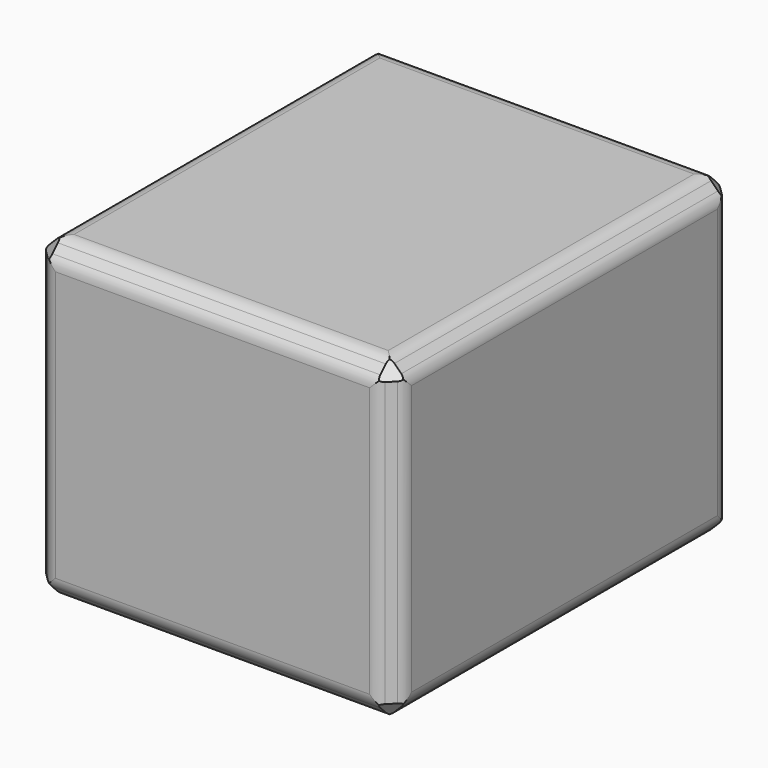
from build123d import *

# Parameters (mm, degrees)
F0_W        = 111.1548654735
F0_H        = 97.4772460759
F1_DEPTH    = 132.08
F2_SIZE     = 5.08
F3_T1_DEPTH = 132.4410244843
F3_T3_DEPTH = 111.5158899578
F3_T5_DEPTH = 97.8382705601


# Not quite as in the source:
# - a fillet or chamfer that OpenCascade refuses, or shapes differently, is made with other operations: its cross-section is extruded or revolved along the edge and cut away or added


with BuildPart() as f1:
    # F0 (on Front) → F1 (new body)
    with BuildSketch(Plane.XZ):
        with Locations((-0.1736786216, 1.3392996043)):
            Rectangle(F0_W, F0_H)
    extrude(amount=F1_DEPTH)

    # F2
    f2_edges = [f1.edges().sort_by_distance(p)[0] for p in [
        (55.403754, -66.04, 50.077923),
        (-55.751111, -66.04, 50.077923),
        (-0.173679, 0, 50.077923),
        (-0.173679, -132.08, 50.077923),
        (55.403754, -66.04, -47.399323),
        (55.403754, 0, 1.3393),
        (55.403754, -132.08, 1.3393),
        (-55.751111, -132.08, 1.3393),
        (-0.173679, -132.08, -47.399323),
        (-55.751111, -66.04, -47.399323),
        (-0.173679, 0, -47.399323),
        (-55.751111, 0, 1.3393),
    ]]
    chamfer(f2_edges, length=F2_SIZE)

    # F3: fillet of radius 5.08 on 24 edges, made by hand

    # F3_s2 → F3_t1 (cut)
    with BuildSketch(Plane.XZ.offset(-0.1805122421)):
        with BuildLine():
            ThreePointArc((48.2195492182, 50.0779226422), (50.1635810547, 49.6912306674), (51.8116516667, 48.5900250907))
            Line((51.8116516667, 48.5900250907), (50.3237541151, 50.0779226422))
            Line((50.3237541151, 50.0779226422), (48.2195492182, 50.0779226422))
        make_face()
        with BuildLine():
            ThreePointArc((-48.5669064615, 50.0779226422), (-50.510938298, 49.6912306674), (-52.15900891, 48.5900250907))
            Line((-52.15900891, 48.5900250907), (-50.6711113584, 50.0779226422))
            Line((-50.6711113584, 50.0779226422), (-48.5669064615, 50.0779226422))
        make_face()
        with BuildLine():
            ThreePointArc((53.9158565635, 46.4858201938), (55.0170621403, 44.8377495818), (55.4037541151, 42.8937177454))
            Line((55.4037541151, 42.8937177454), (55.4037541151, 44.9979226422))
            Line((55.4037541151, 44.9979226422), (53.9158565635, 46.4858201938))
        make_face()
        with BuildLine():
            ThreePointArc((55.4037541151, -40.2151185368), (55.0170621403, -42.1591503732), (53.9158565635, -43.8072209852))
            Line((53.9158565635, -43.8072209852), (55.4037541151, -42.3193234336))
            Line((55.4037541151, -42.3193234336), (55.4037541151, -40.2151185368))
        make_face()
        with BuildLine():
            ThreePointArc((51.8116516667, -45.9114258821), (50.1635810547, -47.0126314588), (48.2195492182, -47.3993234336))
            Line((48.2195492182, -47.3993234336), (50.3237541151, -47.3993234336))
            Line((50.3237541151, -47.3993234336), (51.8116516667, -45.9114258821))
        make_face()
        with BuildLine():
            ThreePointArc((-52.15900891, -45.9114258821), (-50.510938298, -47.0126314588), (-48.5669064615, -47.3993234336))
            Line((-48.5669064615, -47.3993234336), (-50.6711113584, -47.3993234336))
            Line((-50.6711113584, -47.3993234336), (-52.15900891, -45.9114258821))
        make_face()
        with BuildLine():
            ThreePointArc((-54.2632138068, 46.4858201938), (-55.3644193836, 44.8377495818), (-55.7511113584, 42.8937177454))
            Line((-55.7511113584, 42.8937177454), (-55.7511113584, 44.9979226422))
            Line((-55.7511113584, 44.9979226422), (-54.2632138068, 46.4858201938))
        make_face()
        with BuildLine():
            ThreePointArc((-55.7511113584, -40.2151185368), (-55.3644193836, -42.1591503732), (-54.2632138068, -43.8072209852))
            Line((-54.2632138068, -43.8072209852), (-55.7511113584, -42.3193234336))
            Line((-55.7511113584, -42.3193234336), (-55.7511113584, -40.2151185368))
        make_face()
    extrude(amount=F3_T1_DEPTH, mode=Mode.SUBTRACT)

    # F3_s4 → F3_t3 (cut)
    with BuildSketch(Plane.YZ.offset(-55.9316236005)):
        with BuildLine():
            ThreePointArc((-7.1842048969, 50.0779226422), (-5.2401730604, 49.6912306674), (-3.5921024484, 48.5900250907))
            Line((-3.5921024484, 48.5900250907), (-5.08, 50.0779226422))
            Line((-5.08, 50.0779226422), (-7.1842048969, 50.0779226422))
        make_face()
        with BuildLine():
            ThreePointArc((-124.8957951031, 50.0779226422), (-126.8398269396, 49.6912306674), (-128.4878975516, 48.5900250907))
            Line((-128.4878975516, 48.5900250907), (-127, 50.0779226422))
            Line((-127, 50.0779226422), (-124.8957951031, 50.0779226422))
        make_face()
        with BuildLine():
            ThreePointArc((-1.4878975516, 46.4858201938), (-0.3866919748, 44.8377495818), (0, 42.8937177454))
            Line((0, 42.8937177454), (0, 44.9979226422))
            Line((0, 44.9979226422), (-1.4878975516, 46.4858201938))
        make_face()
        with BuildLine():
            ThreePointArc((0, -40.2151185368), (-0.3866919748, -42.1591503732), (-1.4878975516, -43.8072209852))
            Line((-1.4878975516, -43.8072209852), (0, -42.3193234336))
            Line((0, -42.3193234336), (0, -40.2151185368))
        make_face()
        with BuildLine():
            ThreePointArc((-3.5921024484, -45.9114258821), (-5.2401730604, -47.0126314588), (-7.1842048969, -47.3993234336))
            Line((-7.1842048969, -47.3993234336), (-5.08, -47.3993234336))
            Line((-5.08, -47.3993234336), (-3.5921024484, -45.9114258821))
        make_face()
        with BuildLine():
            ThreePointArc((-128.4878975516, -45.9114258821), (-126.8398269396, -47.0126314588), (-124.8957951031, -47.3993234336))
            Line((-124.8957951031, -47.3993234336), (-127, -47.3993234336))
            Line((-127, -47.3993234336), (-128.4878975516, -45.9114258821))
        make_face()
        with BuildLine():
            ThreePointArc((-130.5921024484, 46.4858201938), (-131.6933080252, 44.8377495818), (-132.08, 42.8937177454))
            Line((-132.08, 42.8937177454), (-132.08, 44.9979226422))
            Line((-132.08, 44.9979226422), (-130.5921024484, 46.4858201938))
        make_face()
        with BuildLine():
            ThreePointArc((-132.08, -40.2151185368), (-131.6933080252, -42.1591503732), (-130.5921024484, -43.8072209852))
            Line((-130.5921024484, -43.8072209852), (-132.08, -42.3193234336))
            Line((-132.08, -42.3193234336), (-132.08, -40.2151185368))
        make_face()
    extrude(amount=F3_T3_DEPTH, mode=Mode.SUBTRACT)

    # F3_s6 → F3_t5 (cut)
    with BuildSketch(Plane.XY.offset(-47.5798356758)):
        with BuildLine():
            ThreePointArc((48.2195492182, 0), (50.1635810547, -0.3866919748), (51.8116516667, -1.4878975516))
            Line((51.8116516667, -1.4878975516), (50.3237541151, 0))
            Line((50.3237541151, 0), (48.2195492182, 0))
        make_face()
        with BuildLine():
            ThreePointArc((-48.5669064615, 0), (-50.510938298, -0.3866919748), (-52.15900891, -1.4878975516))
            Line((-52.15900891, -1.4878975516), (-50.6711113584, 0))
            Line((-50.6711113584, 0), (-48.5669064615, 0))
        make_face()
        with BuildLine():
            ThreePointArc((55.4037541151, -7.1842048969), (55.0170621403, -5.2401730604), (53.9158565635, -3.5921024484))
            Line((53.9158565635, -3.5921024484), (55.4037541151, -5.08))
            Line((55.4037541151, -5.08), (55.4037541151, -7.1842048969))
        make_face()
        with BuildLine():
            ThreePointArc((55.4037541151, -124.8957951031), (55.0170621403, -126.8398269396), (53.9158565635, -128.4878975516))
            Line((53.9158565635, -128.4878975516), (55.4037541151, -127))
            Line((55.4037541151, -127), (55.4037541151, -124.8957951031))
        make_face()
        with BuildLine():
            ThreePointArc((-55.7511113584, -7.1842048969), (-55.3644193836, -5.2401730604), (-54.2632138068, -3.5921024484))
            Line((-54.2632138068, -3.5921024484), (-55.7511113584, -5.08))
            Line((-55.7511113584, -5.08), (-55.7511113584, -7.1842048969))
        make_face()
        with BuildLine():
            ThreePointArc((-55.7511113584, -124.8957951031), (-55.3644193836, -126.8398269396), (-54.2632138068, -128.4878975516))
            Line((-54.2632138068, -128.4878975516), (-55.7511113584, -127))
            Line((-55.7511113584, -127), (-55.7511113584, -124.8957951031))
        make_face()
        with BuildLine():
            ThreePointArc((48.2195492182, -132.08), (50.1635810547, -131.6933080252), (51.8116516667, -130.5921024484))
            Line((51.8116516667, -130.5921024484), (50.3237541151, -132.08))
            Line((50.3237541151, -132.08), (48.2195492182, -132.08))
        make_face()
        with BuildLine():
            ThreePointArc((-48.5669064615, -132.08), (-50.510938298, -131.6933080252), (-52.15900891, -130.5921024484))
            Line((-52.15900891, -130.5921024484), (-50.6711113584, -132.08))
            Line((-50.6711113584, -132.08), (-48.5669064615, -132.08))
        make_face()
    extrude(amount=F3_T5_DEPTH, mode=Mode.SUBTRACT)


solid = f1.part
